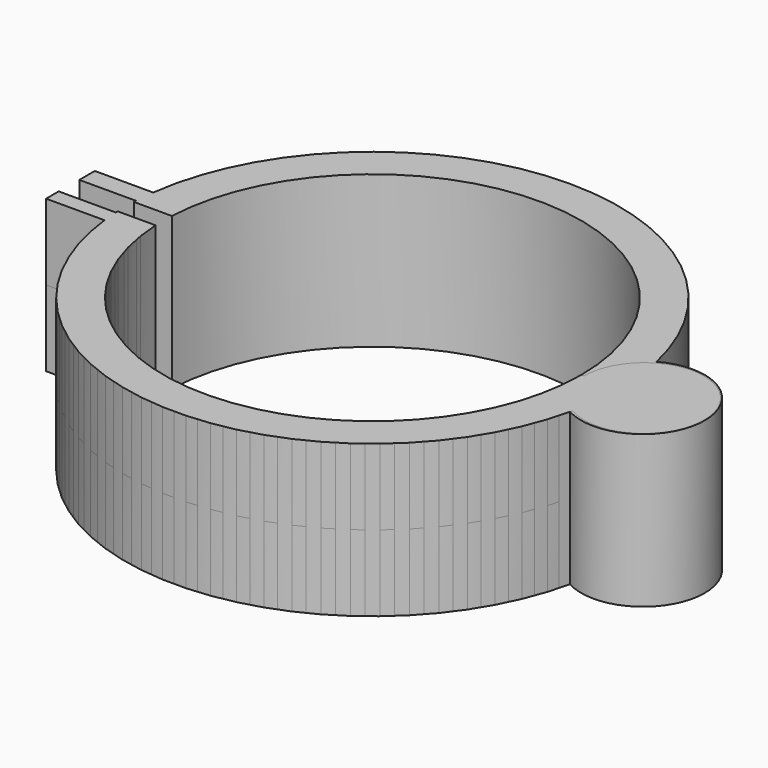
from build123d import *

# Parameters (mm, degrees)
F0_R      = 2.05
F1_DEPTH  = 4
F2_DEPTH  = 2
F5_DEPTH  = 4
F6_W      = 7.8420564532
F6_H      = 1.0693569202
F7_DEPTH  = 4.5
F0_R_2    = 1.7
F8_DEPTH  = 2
F9_DEPTH  = 4
F10_W     = 1.5671141446
F10_H     = 0.3430901561
F11_DEPTH = 4
F12_DEPTH = 4
F13_DEPTH = 4
F14_DEPTH = 4


# Not quite as in the source:
# - the program builds the solid bodies; features that only make, move or delete a surface that nothing else refers to are left out


with BuildPart() as f1:
    # F0 (on Top) → F1 (new body, symmetric)
    with BuildSketch(Plane.XY):
        with BuildLine():
            ThreePointArc((-11, 0), (0, 11), (11, 0))
            ThreePointArc((11, 0), (11.4525622626, 1.6543403837), (12.6842105263, 2.8479472123))
            ThreePointArc((12.6842105263, 2.8479472123), (-0.5898274536, 12.986612475), (-12.8901523849, 1.6864078669))
            Line((-12.8901523849, 1.6864078669), (-12.8901523849, 0.6666785921))
            Line((-12.8901523849, 0.6666785921), (-12.9828941171, 0.6666785921))
            ThreePointArc((-12.9828941171, 0.6666785921), (-12.9957228256, 0.3334490052), (-13, 0))
            Line((-13, 0), (-11, 0))
        make_face()
        with BuildLine():
            ThreePointArc((12.6842105263, 2.8479472123), (11.4525622626, 1.6543403837), (11, 0))
            ThreePointArc((11, 0), (11.4525622626, -1.6543403837), (12.6842105263, -2.8479472123))
            ThreePointArc((12.6842105263, -2.8479472123), (15.9043403837, -2.7974377374), (17.5, 0))
            ThreePointArc((17.5, 0), (15.9043403837, 2.7974377374), (12.6842105263, 2.8479472123))
        make_face()
        with Locations((14.25, 0)):
            Circle(F0_R, mode=Mode.SUBTRACT)
        with BuildLine():
            Line((-12.8901523849, 0.6666785921), (-12.8901523849, 1.6864078669))
            ThreePointArc((-12.8901523849, 1.6864078669), (-12.9465669493, 1.1774566778), (-12.9828941171, 0.6666785921))
            Line((-12.9828941171, 0.6666785921), (-12.8901523849, 0.6666785921))
        make_face()
        with BuildLine():
            ThreePointArc((-12.9828941171, 0.6666785921), (-12.9465669493, 1.1774566778), (-12.8901523849, 1.6864078669))
            Line((-12.8901523849, 1.6864078669), (-15.9636270255, 1.6864078669))
            Line((-15.9636270255, 1.6864078669), (-15.9636270255, 0.6666785921))
            Line((-15.9636270255, 0.6666785921), (-12.9828941171, 0.6666785921))
        make_face()
    extrude(amount=F1_DEPTH, both=True)

    # F0 (on Top) → F2 (cut, symmetric)
    with BuildSketch(Plane.XY):
        with BuildLine():
            ThreePointArc((12.6842105263, 2.8479472123), (11.4525622626, 1.6543403837), (11, 0))
            ThreePointArc((11, 0), (11.4525622626, -1.6543403837), (12.6842105263, -2.8479472123))
            ThreePointArc((12.6842105263, -2.8479472123), (15.9043403837, -2.7974377374), (17.5, 0))
            ThreePointArc((17.5, 0), (15.9043403837, 2.7974377374), (12.6842105263, 2.8479472123))
        make_face()
        with Locations((14.25, 0)):
            Circle(F0_R, mode=Mode.SUBTRACT)
    extrude(amount=F2_DEPTH, both=True, mode=Mode.SUBTRACT)


with BuildPart() as f5:
    # F3 (on Top) → F5 (new body, symmetric)
    with BuildSketch(Plane.XY):
        with BuildLine():
            ThreePointArc((11, 0), (0, -11), (-11, 0))
            Line((-11, 0), (-13, 0))
            ThreePointArc((-13, 0), (-12.9957895083, -0.3308399253), (-12.9831607606, -0.6614655431))
            Line((-12.9831607606, -0.6614655431), (-12.9139886071, -0.6614655431))
            Line((-12.9139886071, -0.6614655431), (-12.9139886071, -1.4929495154))
            ThreePointArc((-12.9139886071, -1.4929495154), (-0.6222206293, -12.98510075), (12.7120691767, -2.7209000803))
            ThreePointArc((12.7120691767, -2.7209000803), (11.5677693449, -1.5688883132), (11.1492688343, 0))
            Line((11.1492688343, 0), (11, 0))
        make_face()
    extrude(amount=F5_DEPTH, both=True)


with BuildPart() as f7_tool:
    # F6 (on Top) → F7 (new body, symmetric)
    with BuildSketch(Plane.XY):
        with Locations((-13.9199756086, 0)):
            Rectangle(F6_W, F6_H)
    extrude(amount=F7_DEPTH, both=True)


with BuildPart() as f1_1:
    add(f1.part)

    # F7: cut by f7_tool
    add(f7_tool.part, mode=Mode.SUBTRACT)


with BuildPart() as f5_1:
    add(f5.part)

    # F7: cut by f7_tool
    add(f7_tool.part, mode=Mode.SUBTRACT)


with BuildPart() as f8:
    # F0 (on Top) → F8 (new body, symmetric)
    with BuildSketch(Plane.XY):
        with Locations((14.25, 0)):
            Circle(F0_R)
        with Locations((14.25, 0)):
            Circle(F0_R_2, mode=Mode.SUBTRACT)
    extrude(amount=F8_DEPTH, both=True)

    # F0 (on Top) → F9 (join, symmetric)
    with BuildSketch(Plane.XY):
        with Locations((14.25, 0)):
            Circle(F0_R_2)
    extrude(amount=F9_DEPTH, both=True)


with BuildPart() as f11_tool:
    # F10 (on Top) → F11 (new body, symmetric)
    with BuildSketch(Plane.XY):
        with Locations((11.4076789469, 0)):
            Rectangle(F10_W, F10_H)
    extrude(amount=F11_DEPTH, both=True)


with BuildPart() as f1_2:
    add(f1_1.part)

    # F11: cut by f11_tool
    add(f11_tool.part, mode=Mode.SUBTRACT)



with BuildPart() as f5_2:
    add(f5_1.part)

    # F11: cut by f11_tool
    add(f11_tool.part, mode=Mode.SUBTRACT)


with BuildPart() as f1_3:
    add(f1_2.part)

    add(f5_2.part)  # F12 merges F5

    add(f8.part)  # F12 merges F8
    # F0 (on Top) → F12 (join, symmetric)
    with BuildSketch(Plane.XY):
        with BuildLine():
            ThreePointArc((-11, 0), (0, 11), (11, 0))
            ThreePointArc((11, 0), (11.4525622626, 1.6543403837), (12.6842105263, 2.8479472123))
            ThreePointArc((12.6842105263, 2.8479472123), (-0.5898274536, 12.986612475), (-12.8901523849, 1.6864078669))
            Line((-12.8901523849, 1.6864078669), (-12.8901523849, 0.6666785921))
            Line((-12.8901523849, 0.6666785921), (-12.9828941171, 0.6666785921))
            ThreePointArc((-12.9828941171, 0.6666785921), (-12.9957228256, 0.3334490052), (-13, 0))
            Line((-13, 0), (-11, 0))
        make_face()
        with BuildLine():
            ThreePointArc((12.6842105263, 2.8479472123), (11.4525622626, 1.6543403837), (11, 0))
            ThreePointArc((11, 0), (11.4525622626, -1.6543403837), (12.6842105263, -2.8479472123))
            ThreePointArc((12.6842105263, -2.8479472123), (15.9043403837, -2.7974377374), (17.5, 0))
            ThreePointArc((17.5, 0), (15.9043403837, 2.7974377374), (12.6842105263, 2.8479472123))
        make_face()
        with Locations((14.25, 0)):
            Circle(F0_R, mode=Mode.SUBTRACT)
        with BuildLine():
            Line((-12.8901523849, 0.6666785921), (-12.8901523849, 1.6864078669))
            ThreePointArc((-12.8901523849, 1.6864078669), (-12.9465669493, 1.1774566778), (-12.9828941171, 0.6666785921))
            Line((-12.9828941171, 0.6666785921), (-12.8901523849, 0.6666785921))
        make_face()
        with BuildLine():
            ThreePointArc((-12.9828941171, 0.6666785921), (-12.9465669493, 1.1774566778), (-12.8901523849, 1.6864078669))
            Line((-12.8901523849, 1.6864078669), (-15.9636270255, 1.6864078669))
            Line((-15.9636270255, 1.6864078669), (-15.9636270255, 0.6666785921))
            Line((-15.9636270255, 0.6666785921), (-12.9828941171, 0.6666785921))
        make_face()
    extrude(amount=F12_DEPTH, both=True)


with BuildPart() as f13:
    # F3 (on Top) → F13 (new body, symmetric)
    with BuildSketch(Plane.XY):
        with BuildLine():
            ThreePointArc((11, 0), (0, -11), (-11, 0))
            Line((-11, 0), (-13, 0))
            ThreePointArc((-13, 0), (-12.9957895083, -0.3308399253), (-12.9831607606, -0.6614655431))
            Line((-12.9831607606, -0.6614655431), (-12.9139886071, -0.6614655431))
            Line((-12.9139886071, -0.6614655431), (-12.9139886071, -1.4929495154))
            ThreePointArc((-12.9139886071, -1.4929495154), (-0.6222206293, -12.98510075), (12.7120691767, -2.7209000803))
            ThreePointArc((12.7120691767, -2.7209000803), (11.5677693449, -1.5688883132), (11.1492688343, 0))
            Line((11.1492688343, 0), (11, 0))
        make_face()
        with BuildLine():
            ThreePointArc((17.4492688343, 0), (14.2992688343, 3.15), (11.1492688343, 0))
            Line((11.1492688343, 0), (13, 0))
            ThreePointArc((13, 0), (12.9278168941, -1.3680461803), (12.7120691767, -2.7209000803))
            ThreePointArc((12.7120691767, -2.7209000803), (15.8681571475, -2.7314994894), (17.4492688343, 0))
        make_face()
        with BuildLine():
            Line((13, 0), (11.1492688343, 0))
            ThreePointArc((11.1492688343, 0), (11.5677693449, -1.5688883132), (12.7120691767, -2.7209000803))
            ThreePointArc((12.7120691767, -2.7209000803), (12.9278168941, -1.3680461803), (13, 0))
        make_face()
        with BuildLine():
            Line((-12.9139886071, -0.6614655431), (-12.9831607606, -0.6614655431))
            ThreePointArc((-12.9831607606, -0.6614655431), (-12.9552471124, -1.0777626166), (-12.9139886071, -1.4929495154))
            Line((-12.9139886071, -1.4929495154), (-12.9139886071, -0.6614655431))
        make_face()
        with BuildLine():
            ThreePointArc((-12.9139886071, -1.4929495154), (-12.9552471124, -1.0777626166), (-12.9831607606, -0.6614655431))
            Line((-12.9831607606, -0.6614655431), (-15.9874632477, -0.6614655431))
            Line((-15.9874632477, -0.6614655431), (-15.9874632477, -1.4929495154))
            Line((-15.9874632477, -1.4929495154), (-12.9139886071, -1.4929495154))
        make_face()
    extrude(amount=F13_DEPTH, both=True)


with BuildPart() as f14_tool:
    # F6 (on Top) → F14 (new body, symmetric)
    with BuildSketch(Plane.XY):
        with Locations((-13.9199756086, 0)):
            Rectangle(F6_W, F6_H)
    extrude(amount=F14_DEPTH, both=True)


with BuildPart() as f1_4:
    add(f1_3.part)

    # F14: cut by f14_tool
    add(f14_tool.part, mode=Mode.SUBTRACT)


with BuildPart() as f13_1:
    add(f13.part)

    # F14: cut by f14_tool
    add(f14_tool.part, mode=Mode.SUBTRACT)


solid = Compound([f1_4.part, f13_1.part])
